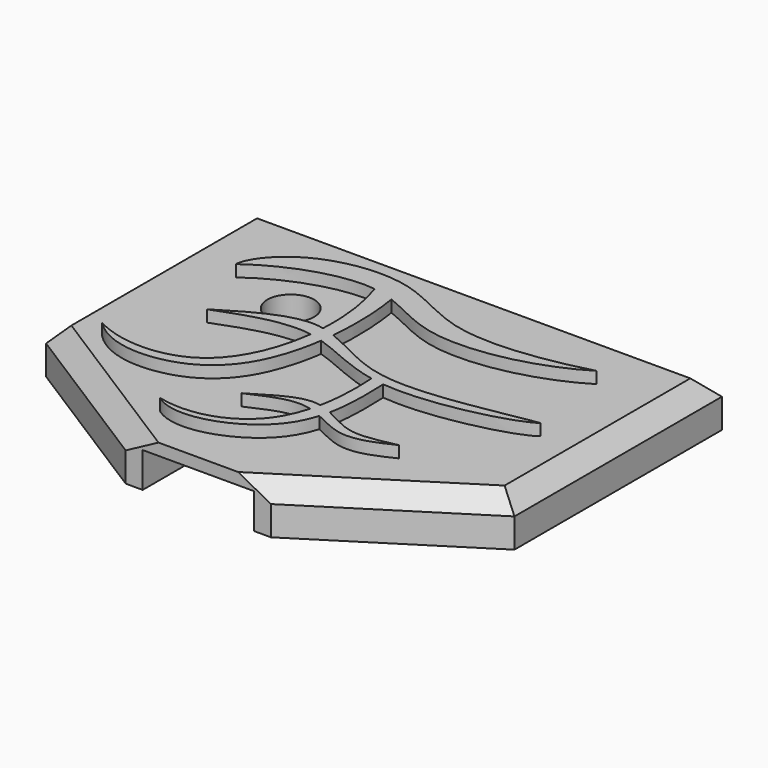
from build123d import *

# Parameters (mm, degrees)
F0_W     = 30
F0_H     = 14.4
F0_W_2   = 9.5
F0_H_2   = 5
F1_DEPTH = 4
F2_DEPTH = 3
F4_DEPTH = 1
F5_SIZE  = 1.5


with BuildPart() as f1:
    # F0 (on Top) → F1 (new body)
    with BuildSketch(Plane.XY):
        Polygon((-43.1869083047, 6.5), (-43.1869083047, 20.9), (-13.1869083047, 20.9), (-13.1869083047, 6.5), (-23.4369083047, 0), (-23.4369083047, -5), (-21.9851882324, -5), (-8.1869083047, 3.7501287347), (-8.1869083047, 25.9), (-48.1869083047, 25.9), (-48.1869083047, 3.7501287347), (-34.388628377, -5), (-32.9369083047, -5), (-32.9369083047, 0), align=None)
        with Locations((-28.1869083047, 13.7)):
            Rectangle(F0_W, F0_H)
        Polygon((-39.1032992899, 13.9), (-39.1032992899, 17.9), (-18.1869083047, 17.9), (-18.1869083047, 13.9), (-28.6451037973, 10.8), align=None, mode=Mode.SUBTRACT)
        Polygon((-13.1869083047, 6.5), (-43.1869083047, 6.5), (-32.9369083047, 0), (-23.4369083047, 0), align=None)
        with Locations((-28.1869083047, -2.5)):
            Rectangle(F0_W_2, F0_H_2)
        with BuildLine():
            Line((-18.1869083047, 17.9), (-39.1032992899, 17.9))
            Line((-39.1032992899, 17.9), (-39.1032992899, 13.9))
            Line((-39.1032992899, 13.9), (-37.7786630825, 13.9))
            ThreePointArc((-37.7786630825, 13.9), (-37.8338156014, 17.3741977051), (-34.8155427277, 15.6528260559))
            ThreePointArc((-34.8155427277, 15.6528260559), (-35.0941710785, 14.6345531822), (-35.8524223729, 13.9))
            Line((-35.8524223729, 13.9), (-18.1869083047, 13.9))
            Line((-18.1869083047, 13.9), (-18.1869083047, 17.9))
        make_face()
        with BuildLine():
            Line((-37.7786630825, 13.9), (-39.1032992899, 13.9))
            Line((-39.1032992899, 13.9), (-28.6451037973, 10.8))
            Line((-28.6451037973, 10.8), (-18.1869083047, 13.9))
            Line((-18.1869083047, 13.9), (-35.8524223729, 13.9))
            ThreePointArc((-35.8524223729, 13.9), (-36.8155427277, 13.6528260559), (-37.7786630825, 13.9))
        make_face()
    extrude(amount=F1_DEPTH)

    # F0 (on Top) → F2 (cut)
    with BuildSketch(Plane.XY):
        with Locations((-28.1869083047, 13.7)):
            Rectangle(F0_W, F0_H)
        Polygon((-39.1032992899, 13.9), (-39.1032992899, 17.9), (-18.1869083047, 17.9), (-18.1869083047, 13.9), (-28.6451037973, 10.8), align=None, mode=Mode.SUBTRACT)
        Polygon((-13.1869083047, 6.5), (-43.1869083047, 6.5), (-32.9369083047, 0), (-23.4369083047, 0), align=None)
        with Locations((-28.1869083047, -2.5)):
            Rectangle(F0_W_2, F0_H_2)
    extrude(amount=F2_DEPTH, mode=Mode.SUBTRACT)

    # F5
    f5_edges = [f1.edges().sort_by_distance(p)[0] for p in [
        (-41.287768, -0.624936, 4),
        (-48.186908, 14.825064, 4),
        (-28.186908, 25.9, 4),
        (-8.186908, 14.825064, 4),
        (-15.086048, -0.624936, 4),
    ]]
    chamfer(f5_edges, length=F5_SIZE)


with BuildPart() as f4:
    # F3 (on face) → F4 (new body)
    with BuildSketch(Plane.XY.offset(4)):
        with BuildLine():
            add(Edge.make_bspline(
                [(-42.4654167145, 16.8494712561), (-39.7938375841, 18.8531576552), (-35.864648273, 20.2127791296), (-32.9948905855, 19.8352541775)],
                knots=[0, 0, 0, 0, 0.3367336674, 0.3367336674, 0.3367336674, 0.3367336674], degree=3))
            add(Edge.make_bspline(
                [(-32.9948905855, 19.8352541775), (-32.3440314578, 19.7496317703), (-31.7476673073, 19.5746541344), (-31.1734072618, 19.3531280695)],
                knots=[0.3367336674, 0.3367336674, 0.3367336674, 0.3367336674, 0.4131046384, 0.4131046384, 0.4131046384, 0.4131046384], degree=3))
            add(Edge.make_bspline(
                [(-31.1734072618, 19.3531280695), (-29.5978329229, 18.7453358574), (-25.6508147134, 16.0615042571), (-17.7608904848, 17.5646834939), (-14.0538355336, 19.8352541775)],
                knots=[0.4131046384, 0.4131046384, 0.4131046384, 0.4131046384, 0.6226406196, 1, 1, 1, 1], degree=3))
            add(Edge.make_bspline(
                [(-42.4654167145, 16.8494712561), (-42.3726604929, 18.008949951), (-39.5993766245, 21.4286085388), (-31.3253802251, 22.5074804398), (-25.4250962682, 17.798905064), (-17.9107243535, 18.8059261112), (-14.0538355336, 19.8352541775)],
                knots=[0, 0, 0, 0, 0.1986315254, 0.4523082805, 0.6948192618, 1, 1, 1, 1], degree=3))
        make_face()
        with BuildLine():
            add(Edge.make_bspline(
                [(-32.9948905855, 19.8352541775), (-32.3440314578, 19.7496317703), (-31.7476673073, 19.5746541344), (-31.1734072618, 19.3531280695)],
                knots=[0.3367336674, 0.3367336674, 0.3367336674, 0.3367336674, 0.4131046384, 0.4131046384, 0.4131046384, 0.4131046384], degree=3))
            add(Edge.make_bspline(
                [(-32.9948905855, 19.8352541775), (-32.2896273329, 17.753049629), (-32.0126127544, 15.4491126865), (-32.1345889722, 13.255812889)],
                knots=[0, 0, 0, 0, 0.2225431575, 0.2225431575, 0.2225431575, 0.2225431575], degree=3))
            add(Edge.make_bspline(
                [(-32.134588974, 13.2558128888), (-31.7475533394, 13.1731038166), (-31.3627928139, 13.0483545557), (-30.9761098202, 12.8961333799)],
                knots=[0.3286914696, 0.3286914696, 0.3286914696, 0.3286914696, 0.3802894739, 0.3802894739, 0.3802894739, 0.3802894739], degree=3))
            add(Edge.make_bspline(
                [(-30.976109827, 12.8961333789), (-30.7712879528, 14.9993919589), (-30.8365034569, 17.2432759127), (-31.1734072618, 19.3531280695)],
                knots=[0.8062718014, 0.8062718014, 0.8062718014, 0.8062718014, 1, 1, 1, 1], degree=3))
        make_face()
        with BuildLine():
            add(Edge.make_bspline(
                [(-32.1345889722, 13.255812889), (-32.1569847951, 12.8531052564), (-32.1928313712, 12.4541274165), (-32.2419476004, 12.0609366653)],
                knots=[0.2225431575, 0.2225431575, 0.2225431575, 0.2225431575, 0.2634038863, 0.2634038863, 0.2634038863, 0.2634038863], degree=3))
            add(Edge.make_bspline(
                [(-39.8995094001, 10.551338084), (-37.4732565623, 12.0421009296), (-34.8160280141, 13.6831493791), (-32.3427257342, 13.3002914763), (-32.134588974, 13.2558128888)],
                knots=[0, 0, 0, 0, 0.3009435298, 0.3286914696, 0.3286914696, 0.3286914696, 0.3286914696], degree=3))
            add(Edge.make_bspline(
                [(-39.8995094001, 10.551338084), (-38.2007072715, 11.1867110314), (-35.0695646892, 12.456761007), (-32.4286591287, 12.094066028), (-32.2419476145, 12.0609366664)],
                knots=[0, 0, 0, 0, 0.2934865557, 0.3160525993, 0.3160525993, 0.3160525993, 0.3160525993], degree=3))
        make_face()
        with BuildLine():
            add(Edge.make_bspline(
                [(-30.9761098202, 12.8961333799), (-29.2963172809, 12.23486821), (-24.551812522, 8.9733096857), (-16.899658367, 10.8779082075), (-12.2810266912, 11.6243530065)],
                knots=[0.3802894739, 0.3802894739, 0.3802894739, 0.3802894739, 0.6044367579, 1, 1, 1, 1], degree=3))
            add(Edge.make_bspline(
                [(-31.112915177, 11.7758911415), (-31.0585745099, 12.1436838454), (-31.0129695193, 12.5176314999), (-30.976109827, 12.8961333789)],
                knots=[0.771408524, 0.771408524, 0.771408524, 0.771408524, 0.8062718014, 0.8062718014, 0.8062718014, 0.8062718014], degree=3))
            add(Edge.make_bspline(
                [(-31.1129151777, 11.7758911415), (-29.2735553981, 11.1875546271), (-27.486927637, 10.0877460543), (-25.0796457725, 9.6045233315)],
                knots=[0.362248868, 0.362248868, 0.362248868, 0.362248868, 0.590469567, 0.590469567, 0.590469567, 0.590469567], degree=3))
            add(Edge.make_bspline(
                [(-25.0796457725, 9.6045233315), (-24.7161044464, 9.5315483168), (-24.3384083341, 9.4726353068), (-23.9442382008, 9.4316694885)],
                knots=[0.590469567, 0.590469567, 0.590469567, 0.590469567, 0.624934852, 0.624934852, 0.624934852, 0.624934852], degree=3))
            add(Edge.make_bspline(
                [(-23.9442382008, 9.4316694885), (-19.6547196513, 8.985862913), (-13.4142369665, 10.665483242), (-12.2810266912, 11.6243530065)],
                knots=[0.624934852, 0.624934852, 0.624934852, 0.624934852, 1, 1, 1, 1], degree=3))
        make_face()
        with BuildLine():
            add(Edge.make_bspline(
                [(-32.134588974, 13.2558128888), (-31.7475533394, 13.1731038166), (-31.3627928139, 13.0483545557), (-30.9761098202, 12.8961333799)],
                knots=[0.3286914696, 0.3286914696, 0.3286914696, 0.3286914696, 0.3802894739, 0.3802894739, 0.3802894739, 0.3802894739], degree=3))
            add(Edge.make_bspline(
                [(-32.1345889722, 13.255812889), (-32.1569847951, 12.8531052564), (-32.1928313712, 12.4541274165), (-32.2419476004, 12.0609366653)],
                knots=[0.2225431575, 0.2225431575, 0.2225431575, 0.2225431575, 0.2634038863, 0.2634038863, 0.2634038863, 0.2634038863], degree=3))
            add(Edge.make_bspline(
                [(-32.2419476145, 12.0609366664), (-31.8597195461, 11.9931156113), (-31.4852370526, 11.8949817928), (-31.1129151777, 11.7758911415)],
                knots=[0.3160525993, 0.3160525993, 0.3160525993, 0.3160525993, 0.362248868, 0.362248868, 0.362248868, 0.362248868], degree=3))
            add(Edge.make_bspline(
                [(-31.112915177, 11.7758911415), (-31.0585745099, 12.1436838454), (-31.0129695193, 12.5176314999), (-30.976109827, 12.8961333789)],
                knots=[0.771408524, 0.771408524, 0.771408524, 0.771408524, 0.8062718014, 0.8062718014, 0.8062718014, 0.8062718014], degree=3))
        make_face()
        with BuildLine():
            add(Edge.make_bspline(
                [(-32.2419476145, 12.0609366664), (-31.8597195461, 11.9931156113), (-31.4852370526, 11.8949817928), (-31.1129151777, 11.7758911415)],
                knots=[0.3160525993, 0.3160525993, 0.3160525993, 0.3160525993, 0.362248868, 0.362248868, 0.362248868, 0.362248868], degree=3))
            add(Edge.make_bspline(
                [(-32.2419476004, 12.0609366653), (-32.6073918669, 9.1354412048), (-35.2726418826, 2.8236045142), (-41.8122783303, 3.3667995594), (-44.1449210048, 4.6730795875)],
                knots=[0.2634038863, 0.2634038863, 0.2634038863, 0.2634038863, 0.5674239482, 1, 1, 1, 1], degree=3))
            add(Edge.make_bspline(
                [(-44.1449210048, 4.6730795875), (-42.4360304347, 2.9172204585), (-37.6356661883, 2.2588303615), (-32.7788568242, 5.2397269583), (-31.4013304686, 9.8238164685), (-31.112915177, 11.7758911415)],
                knots=[0, 0, 0, 0, 0.2945227107, 0.5863702675, 0.771408524, 0.771408524, 0.771408524, 0.771408524], degree=3))
        make_face()
        with BuildLine():
            add(Edge.make_bspline(
                [(-25.0796457725, 9.6045233315), (-24.7161044464, 9.5315483168), (-24.3384083341, 9.4726353068), (-23.9442382008, 9.4316694885)],
                knots=[0.590469567, 0.590469567, 0.590469567, 0.590469567, 0.624934852, 0.624934852, 0.624934852, 0.624934852], degree=3))
            add(Edge.make_bspline(
                [(-25.0796457725, 9.6045233315), (-24.9734072616, 8.0267808085), (-24.9890853523, 6.1789301298), (-25.3412728696, 4.4612159346)],
                knots=[0, 0, 0, 0, 0.2932023186, 0.2932023186, 0.2932023186, 0.2932023186], degree=3))
            add(Edge.make_bspline(
                [(-25.3412728564, 4.4612159321), (-24.9556596717, 4.3763306971), (-24.5736644604, 4.2275105969), (-24.197272273, 4.053112762)],
                knots=[0.3940903335, 0.3940903335, 0.3940903335, 0.3940903335, 0.486042244, 0.486042244, 0.486042244, 0.486042244], degree=3))
            add(Edge.make_bspline(
                [(-23.9442382008, 9.4316694885), (-23.8685441759, 7.5140960035), (-23.8520826412, 5.6859897217), (-24.1972722811, 4.053112762)],
                knots=[0, 0, 0, 0, 0.2764976522, 0.2764976522, 0.2764976522, 0.2764976522], degree=3))
        make_face()
        with BuildLine():
            add(Edge.make_bspline(
                [(-24.197272273, 4.053112762), (-23.4309801461, 3.6980584003), (-21.3909257082, 2.4322158399), (-19.6521766484, 2.8069657274), (-17.6461040974, 3.2268413343)],
                knots=[0.486042244, 0.486042244, 0.486042244, 0.486042244, 0.6732459838, 1, 1, 1, 1], degree=3))
            add(Edge.make_bspline(
                [(-24.1972722811, 4.053112762), (-24.258280878, 3.7645191292), (-24.3305863011, 3.482023836), (-24.4158581353, 3.2062107713)],
                knots=[0.2764976522, 0.2764976522, 0.2764976522, 0.2764976522, 0.325365671, 0.325365671, 0.325365671, 0.325365671], degree=3))
            add(Edge.make_bspline(
                [(-24.4158581101, 3.2062107668), (-23.590972038, 2.8311126201), (-21.4214831622, 1.6170506773), (-19.3722583354, 2.3870898876), (-17.6461040974, 3.2268413343)],
                knots=[0.4686999018, 0.4686999018, 0.4686999018, 0.4686999018, 0.6674310157, 1, 1, 1, 1], degree=3))
        make_face()
        with BuildLine():
            add(Edge.make_bspline(
                [(-25.3412728564, 4.4612159321), (-24.9556596717, 4.3763306971), (-24.5736644604, 4.2275105969), (-24.197272273, 4.053112762)],
                knots=[0.3940903335, 0.3940903335, 0.3940903335, 0.3940903335, 0.486042244, 0.486042244, 0.486042244, 0.486042244], degree=3))
            add(Edge.make_bspline(
                [(-25.3412728696, 4.4612159346), (-25.3986905319, 4.1811743976), (-25.4650523701, 3.9045917937), (-25.5412882704, 3.6332024867)],
                knots=[0.2932023186, 0.2932023186, 0.2932023186, 0.2932023186, 0.341003535, 0.341003535, 0.341003535, 0.341003535], degree=3))
            add(Edge.make_bspline(
                [(-25.541288286, 3.6332024911), (-25.1636236146, 3.5288828613), (-24.7883749037, 3.375604291), (-24.4158581101, 3.2062107668)],
                knots=[0.3789533539, 0.3789533539, 0.3789533539, 0.3789533539, 0.4686999018, 0.4686999018, 0.4686999018, 0.4686999018], degree=3))
            add(Edge.make_bspline(
                [(-24.1972722811, 4.053112762), (-24.258280878, 3.7645191292), (-24.3305863011, 3.482023836), (-24.4158581353, 3.2062107713)],
                knots=[0.2764976522, 0.2764976522, 0.2764976522, 0.2764976522, 0.325365671, 0.325365671, 0.325365671, 0.325365671], degree=3))
        make_face()
        with BuildLine():
            add(Edge.make_bspline(
                [(-25.3412728696, 4.4612159346), (-25.3986905319, 4.1811743976), (-25.4650523701, 3.9045917937), (-25.5412882704, 3.6332024867)],
                knots=[0.2932023186, 0.2932023186, 0.2932023186, 0.2932023186, 0.341003535, 0.341003535, 0.341003535, 0.341003535], degree=3))
            add(Edge.make_bspline(
                [(-30.5222887546, 2.5270488113), (-28.8819089365, 3.4958588937), (-27.1720866653, 4.7410257623), (-25.5125274132, 4.4989142885), (-25.3412728564, 4.4612159321)],
                knots=[0, 0, 0, 0, 0.3532535978, 0.3940903335, 0.3940903335, 0.3940903335, 0.3940903335], degree=3))
            add(Edge.make_bspline(
                [(-30.5222887546, 2.5270488113), (-28.9472388962, 3.2456805901), (-27.3074611458, 4.0284117853), (-25.7082677545, 3.6793260437), (-25.541288286, 3.6332024911)],
                knots=[0, 0, 0, 0, 0.3392730978, 0.3789533539, 0.3789533539, 0.3789533539, 0.3789533539], degree=3))
        make_face()
        with BuildLine():
            add(Edge.make_bspline(
                [(-25.541288286, 3.6332024911), (-25.1636236146, 3.5288828613), (-24.7883749037, 3.375604291), (-24.4158581101, 3.2062107668)],
                knots=[0.3789533539, 0.3789533539, 0.3789533539, 0.3789533539, 0.4686999018, 0.4686999018, 0.4686999018, 0.4686999018], degree=3))
            add(Edge.make_bspline(
                [(-25.5412882704, 3.6332024867), (-25.8154404803, 2.6572583722), (-27.3559647856, -0.8266993526), (-31.4086936414, -2.1382363047), (-34.347821027, -1.3917906908)],
                knots=[0.341003535, 0.341003535, 0.341003535, 0.341003535, 0.5129016702, 1, 1, 1, 1], degree=3))
            add(Edge.make_bspline(
                [(-24.4158581353, 3.2062107713), (-24.7402109886, 2.1570864562), (-26.5982963118, -1.2996818857), (-32.1379193429, -3.0596398465), (-34.347821027, -1.3917906908)],
                knots=[0.325365671, 0.325365671, 0.325365671, 0.325365671, 0.511247463, 1, 1, 1, 1], degree=3))
        make_face()
    extrude(amount=F4_DEPTH)


solid = Compound([f1.part, f4.part])
